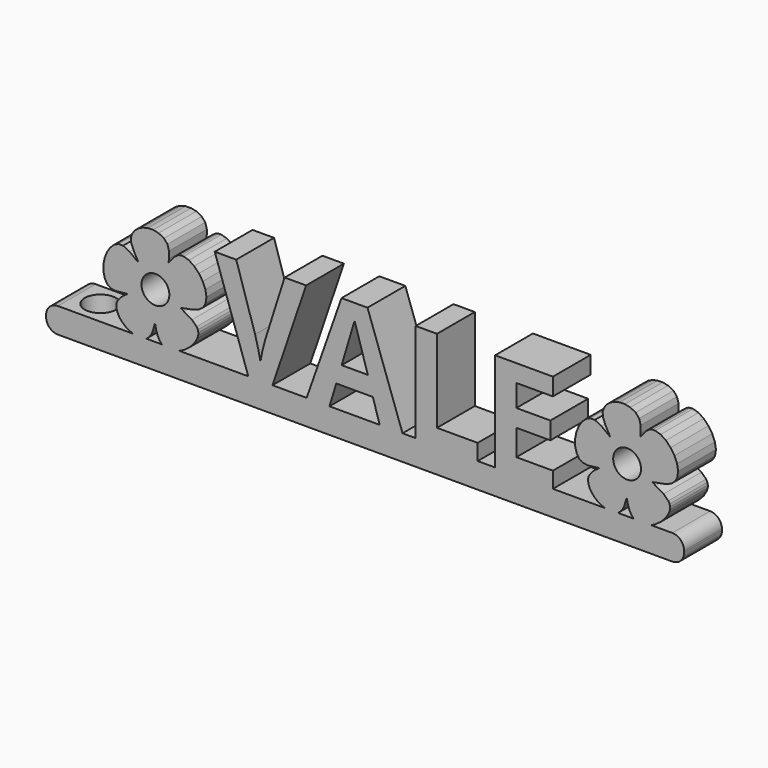
from build123d import *

# Parameters (mm, degrees)
F0_R         = 1.7660260944
F0_TEXT_SIZE = 17.8452958992
F1_DEPTH     = 3
F2_W         = 73.5
F2_H         = 6
F3_DEPTH     = 0.2
F4_DEPTH     = 3
F5_W         = 6
F5_H         = 3.2
F6_DEPTH     = 7.5
F7_R         = 1.5
F8_R         = 2
F9_DEPTH     = 4
F10_R        = 1.5


# Not quite as in the source:
# - Text() gives the source's letters only with a copy of the font that has no kerning and outlines rounded to 1/6400 em; it was checked with that copy


with BuildPart() as f1:
    # F0 (on Front) → F1 (new body, symmetric)
    with BuildSketch(Plane.XZ):
        Polygon((-9.8962181259, -0.0299609487), (-9.3093152472, 0.0995427735), (-8.5310452338, 0.4643787281), (-7.7886221935, 1.0156229815), (-7.1753136859, 1.6703047867), (-6.7844076966, 2.345448762), (-6.6844409889, 2.697736103), (-6.6652413988, 3.0240118702), (-6.7312263226, 3.3305926174), (-6.8868132072, 3.6238062576), (-7.4844896445, 4.1953846804), (-8.4936258745, 4.789299945), (-8.9274018823, 5.0567831788), (-8.4181052429, 5.1580766137), (-7.3131137554, 5.3695361907), (-6.5480905692, 5.6521941874), (-6.0523445823, 6.043851435), (-5.7552051187, 6.5823041299), (-5.6420905942, 7.3346827833), (-5.7751165223, 8.1369112107), (-6.1089634595, 8.9328581362), (-6.5983028952, 9.6663968681), (-7.1978267956, 10.281407439), (-7.8622157172, 10.7217585729), (-8.546147975, 10.9313258196), (-8.8812811082, 10.9320270148), (-9.2043064176, 10.8539824368), (-9.6469000392, 10.5612860557), (-10.1400767255, 9.9810366231), (-10.4508130024, 9.5801644376), (-10.4068223535, 10.0271686751), (-10.3916193646, 10.9311557532), (-10.598433195, 11.6324207168), (-11.0363252865, 12.1480644274), (-11.7143548393, 12.4951945719), (-12.3982545289, 12.6383143795), (-13.0712303381, 12.6247535348), (-13.7032208938, 12.4733707309), (-14.2641853, 12.2030313855), (-14.7240621838, 11.8325941916), (-15.0528129411, 11.3809291004), (-15.2203761991, 10.8668948051), (-15.1967042361, 10.3093544817), (-14.8286469794, 9.4077545862), (-14.3529716358, 8.5454741101), (-14.2906102139, 8.4004774316), (-14.4811582303, 8.5293860258), (-15.3946726039, 9.2300894295), (-16.21802192, 9.6332437342), (-16.8030362894, 9.634121823), (-17.3568401554, 9.3699870508), (-17.8525159958, 8.8932532172), (-18.2631576982, 8.2563454299), (-18.5618432066, 7.5116797807), (-18.7216618753, 6.7116836696), (-18.7156984739, 5.9087754295), (-18.5170445979, 5.1553756349), (-18.2008868091, 4.6439944488), (-17.7512302174, 4.3560670179), (-17.1086136552, 4.2712956407), (-16.2135760559, 4.3694053341), (-15.7044514474, 4.4302814773), (-15.6696932647, 4.4000047008), (-15.7790195709, 4.3290260096), (-16.1651405309, 4.0708069691), (-16.5523139664, 3.7127982689), (-16.8671052824, 3.3322639471), (-17.0360798838, 3.0064680418), (-17.0831036318, 2.6043628391), (-17.0239245605, 2.1921008316), (-16.867618816, 1.7819255621), (-16.6232807801, 1.3860941234), (-16.3000002503, 1.0168545414), (-15.9068693162, 0.6864593752), (-15.4529754831, 0.4071521172), (-14.9474063577, 0.1911989779), (-14.4397479673, 0.0570083052), (-13.9840845603, 0.0188926715), (-13.5797273957, 0.0772799851), (-13.2259605822, 0.2326232662), (-12.9220907946, 0.485341356), (-12.6674066752, 0.8358849825), (-12.4612081239, 1.2846821047), (-12.3027905578, 1.8321743328), (-12.1879723822, 2.2557758958), (-12.1309056827, 2.0998483864), (-12.0112204133, 1.5291342486), (-11.8237778137, 0.9902805659), (-11.5954117235, 0.5466869075), (-11.3529559319, 0.2617414835), (-10.9521058183, 0.053843468), (-10.4551700276, -0.0442881949), align=None)
        with Locations((-12.1185852993, 6.0541479067)):
            Circle(F0_R, mode=Mode.SUBTRACT)
        Polygon((49.7433384922, 9.9810366231), (49.4326022154, 9.5801644376), (49.4765928642, 10.0271686751), (49.4917958531, 10.9311557532), (49.2849820227, 11.6324207168), (48.8470899313, 12.1480644274), (48.1690603785, 12.4951945719), (47.4851606888, 12.6383143795), (46.8121848797, 12.6247535348), (46.180194324, 12.4733707309), (45.6192299178, 12.2030313855), (45.159353034, 11.8325941916), (44.8306022766, 11.3809291004), (44.6630390186, 10.8668948051), (44.6867109816, 10.3093544817), (45.0547682383, 9.4077545862), (45.5304435819, 8.5454741101), (45.5928050038, 8.4004774316), (45.4022569875, 8.5293860258), (44.4887426139, 9.2300894295), (43.6653932978, 9.6332437342), (43.0803789284, 9.634121823), (42.5265750624, 9.3699870508), (42.0308992219, 8.8932532172), (41.6202575196, 8.2563454299), (41.3215720111, 7.5116797807), (41.1617533425, 6.7116836696), (41.1677167439, 5.9087754295), (41.3663706199, 5.1553756349), (41.6825284087, 4.6439944488), (42.1321850004, 4.3560670179), (42.7748015626, 4.2712956407), (43.6698391619, 4.3694053341), (44.1789637704, 4.4302814773), (44.2137219531, 4.4000047008), (44.1043956469, 4.3290260096), (43.7182746869, 4.0708069691), (43.3311012514, 3.7127982689), (43.0163099354, 3.3322639471), (42.847335334, 3.0064680418), (42.8003115859, 2.6043628391), (42.8594906573, 2.1921008316), (43.0157964017, 1.7819255621), (43.2601344376, 1.3860941234), (43.5834149674, 1.0168545414), (43.9765459016, 0.6864593752), (44.4304397347, 0.4071521172), (44.9360088601, 0.1911989779), (45.4436672504, 0.0570083052), (45.8993306575, 0.0188926715), (46.303687822, 0.0772799851), (46.6574546356, 0.2326232662), (46.9613244231, 0.485341356), (47.2160085425, 0.8358849825), (47.4222070939, 1.2846821047), (47.58062466, 1.8321743328), (47.6954428355, 2.2557758958), (47.752509535, 2.0998483864), (47.8721948044, 1.5291342486), (48.059637404, 0.9902805659), (48.2880034942, 0.5466869075), (48.5304592859, 0.2617414835), (48.9313093995, 0.053843468), (49.4282451902, -0.0442881949), (49.9871970919, -0.0299609487), (50.5740999706, 0.0995427735), (51.352369984, 0.4643787281), (52.0947930243, 1.0156229815), (52.7081015319, 1.6703047867), (53.0990075212, 2.345448762), (53.1989742289, 2.697736103), (53.2181738189, 3.0240118702), (53.1521888951, 3.3305926174), (52.9966020106, 3.6238062576), (52.3989255733, 4.1953846804), (51.3897893432, 4.789299945), (50.9560133355, 5.0567831788), (51.4653099749, 5.1580766137), (52.5703014624, 5.3695361907), (53.3353246485, 5.6521941874), (53.8310706354, 6.043851435), (54.128210099, 6.5823041299), (54.2413246235, 7.3346827833), (54.1082986954, 8.1369112107), (53.7744517583, 8.9328581362), (53.2851123226, 9.6663968681), (52.6855884222, 10.281407439), (52.0211995006, 10.7217585729), (51.3372672428, 10.9313258196), (51.0021341095, 10.9320270148), (50.6791088002, 10.8539824368), (50.2365151785, 10.5612860557), align=None)
        with Locations((47.7648299184, 6.0541479067)):
            Circle(F0_R, mode=Mode.SUBTRACT)
        with Locations((-4.589034181, 0)):
            Text('VALE', F0_TEXT_SIZE, font='Open Sans', font_style=FontStyle.BOLD, text_align=(TextAlign.LEFT, TextAlign.BOTTOM))
    extrude(amount=F1_DEPTH, both=True)



with BuildPart() as f3:
    # F2 (on Top) → F3 (new body)
    with BuildSketch(Plane.XY):
        with Locations((18.25, 0)):
            Rectangle(F2_W, F2_H)
    extrude(amount=F3_DEPTH)


with BuildPart() as f4:
    # F4 (new): a face of the model
    f4_faces = [f3.part.faces().sort_by_distance(p)[0] for p in [
        (18.25, 0, 0),
    ]]
    extrude(f4_faces, amount=F4_DEPTH)


with BuildPart() as f1_1:
    add(f1.part)

    add(f3.part)  # F6 merges F3

    add(f4.part)  # F6 merges F4
    # F5 (on face) → F6 (join)
    with BuildSketch(Plane(origin=(-18.5, 0, 0), x_dir=(0, -1, 0), z_dir=(-1, 0, 0))):
        with Locations((0, -1.4)):
            Rectangle(F5_W, F5_H)
    extrude(amount=F6_DEPTH)

    # F7
    f7_edges = [f1_1.edges().sort_by_distance(p)[0] for p in [
        (-26, 0, -3),
        (-26, 0, 0.2),
        (55, 0, -3),
    ]]
    fillet(f7_edges, radius=F7_R)

    # F8 (on face) → F9 (cut)
    with BuildSketch(Plane.XY.offset(0.2)):
        with Locations((-21.5, 0)):
            Circle(F8_R)
    extrude(amount=-F9_DEPTH, mode=Mode.SUBTRACT)

    # F10
    f10_edges = [f1_1.edges().sort_by_distance(p)[0] for p in [
        (55, 0, 0.2),
    ]]
    fillet(f10_edges, radius=F10_R)


solid = f1_1.part
